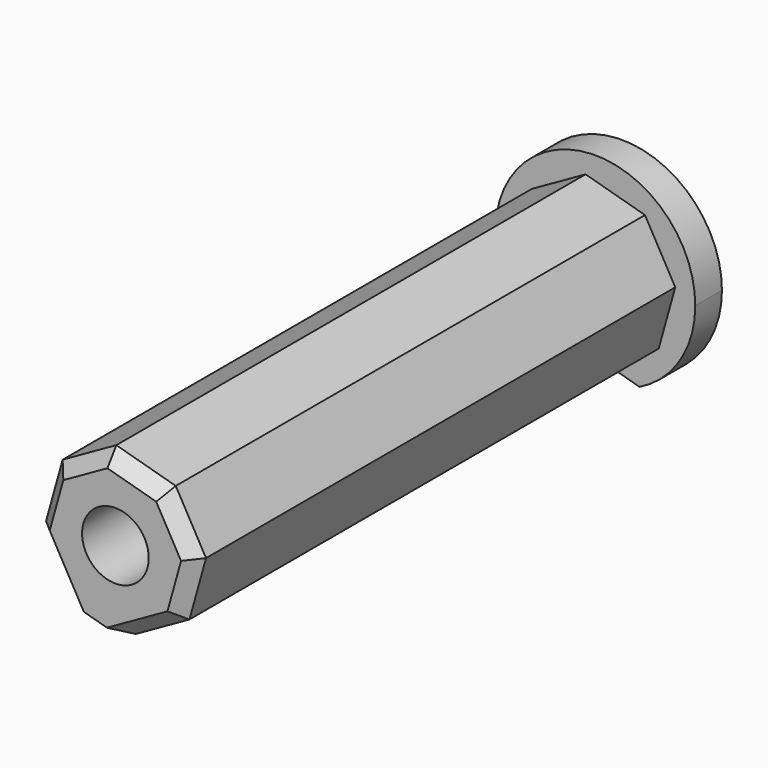
from build123d import *

# Parameters (mm, degrees)
F0_R         = 0.5
F1_DEPTH     = 9
F2_T1_DEPTH  = 1.9538472674
F2_T3_DEPTH  = 1.9538472674
F2_T5_DEPTH  = 1.9538472674
F2_T7_DEPTH  = 1.9538472674
F2_T9_DEPTH  = 1.9538472674
F2_T11_DEPTH = 1.9538472674
F2_T13_DEPTH = 1.9538472674
F3_DEPTH     = 0.5


# Not quite as in the source:
# - a fillet or chamfer that OpenCascade refuses, or shapes differently, is made with other operations: its cross-section is extruded or revolved along the edge and cut away or added


with BuildPart() as f1:
    # F0 (on Front) → F1 (new body)
    with BuildSketch(Plane.XZ):
        Polygon((1.2, 0.1455782856), (0.7455887445, 0.9514675304), (-0.1455782856, 1.2), (-0.9514675304, 0.7455887445), (-1.2, -0.1455782856), (-0.7455887445, -0.9514675304), (0.1455782856, -1.2), (0.9514675304, -0.7455887445), align=None)
        Circle(F0_R, mode=Mode.SUBTRACT)
    extrude(amount=F1_DEPTH)

    # F2: chamfer of 0.2 on 8 edges, made by hand

    # F2_s2 → F2_t1 (cut)
    with BuildSketch(Plane(origin=(0.8509666159, 0, 0.4798287244), x_dir=(0, 1, 0), z_dir=(-0.871067693, 0, -0.4911629813))):
        Polygon((-8.8, -1.1167838964), (-9, -0.9167838964), (-9, -1.1167838964), align=None)
    extrude(amount=F2_T1_DEPTH, mode=Mode.SUBTRACT)

    # F2_s4 → F2_t3 (cut)
    with BuildSketch(Plane(origin=(0.2624341198, 0, 0.9410144095), x_dir=(0, 1, 0), z_dir=(-0.2686331979, 0, -0.9632425473))):
        Polygon((-8.8, -1.1167838964), (-9, -0.9167838964), (-9, -1.1167838964), align=None)
    extrude(amount=F2_T3_DEPTH, mode=Mode.SUBTRACT)

    # F2_s6 → F2_t5 (cut)
    with BuildSketch(Plane(origin=(-0.4798287244, 0, 0.8509666159), x_dir=(0, 1, 0), z_dir=(0.4911629813, 0, -0.871067693))):
        Polygon((-8.8, -1.1167838964), (-9, -0.9167838964), (-9, -1.1167838964), align=None)
    extrude(amount=F2_T5_DEPTH, mode=Mode.SUBTRACT)

    # F2_s8 → F2_t7 (cut)
    with BuildSketch(Plane(origin=(-0.8509666159, 0, -0.4798287244), x_dir=(0, 1, 0), z_dir=(0.871067693, 0, 0.4911629813))):
        Polygon((-8.8, -1.1167838964), (-9, -0.9167838964), (-9, -1.1167838964), align=None)
    extrude(amount=F2_T7_DEPTH, mode=Mode.SUBTRACT)

    # F2_s10 → F2_t9 (cut)
    with BuildSketch(Plane(origin=(-0.2624341198, 0, -0.9410144095), x_dir=(0, 1, 0), z_dir=(0.2686331979, 0, 0.9632425473))):
        Polygon((-8.8, -1.1167838964), (-9, -0.9167838964), (-9, -1.1167838964), align=None)
    extrude(amount=F2_T9_DEPTH, mode=Mode.SUBTRACT)

    # F2_s12 → F2_t11 (cut)
    with BuildSketch(Plane(origin=(0.4798287244, 0, -0.8509666159), x_dir=(0, 1, 0), z_dir=(-0.4911629813, 0, 0.871067693))):
        Polygon((-8.8, -1.1167838964), (-9, -0.9167838964), (-9, -1.1167838964), align=None)
    extrude(amount=F2_T11_DEPTH, mode=Mode.SUBTRACT)

    # F2_s14 → F2_t13 (cut)
    with BuildSketch(Plane(origin=(0.9410144095, 0, -0.2624341198), x_dir=(0, 1, 0), z_dir=(-0.9632425473, 0, 0.2686331979))):
        Polygon((-8.8, -1.1167838964), (-9, -0.9167838964), (-9, -1.1167838964), align=None)
    extrude(amount=F2_T13_DEPTH, mode=Mode.SUBTRACT)

    # F0 (on Front) → F3 (join)
    with BuildSketch(Plane.XZ):
        with BuildLine():
            Line((-0.1455782856, 1.2), (0.7455887445, 0.9514675304))
            Line((0.7455887445, 0.9514675304), (1.2, 0.1455782856))
            Line((1.2, 0.1455782856), (0.9514675304, -0.7455887445))
            Line((0.9514675304, -0.7455887445), (0.1455782856, -1.2))
            Line((0.1455782856, -1.2), (0.6645818987, -1.3447419455))
            ThreePointArc((0.6645818987, -1.3447419455), (1.2741414458, -0.7915576896), (1.5, 0))
            ThreePointArc((1.5, 0), (-0.4201853542, 1.4399459254), (-1.2645923575, -0.8067255849))
            Line((-1.2645923575, -0.8067255849), (-0.7455887445, -0.9514675304))
            Line((-0.7455887445, -0.9514675304), (-1.2, -0.1455782856))
            Line((-1.2, -0.1455782856), (-0.9514675304, 0.7455887445))
            Line((-0.9514675304, 0.7455887445), (-0.1455782856, 1.2))
        make_face()
        Polygon((1.2, 0.1455782856), (0.7455887445, 0.9514675304), (-0.1455782856, 1.2), (-0.9514675304, 0.7455887445), (-1.2, -0.1455782856), (-0.7455887445, -0.9514675304), (0.1455782856, -1.2), (0.9514675304, -0.7455887445), align=None)
        Circle(F0_R, mode=Mode.SUBTRACT)
        Circle(F0_R)
    extrude(amount=-F3_DEPTH)


solid = f1.part
